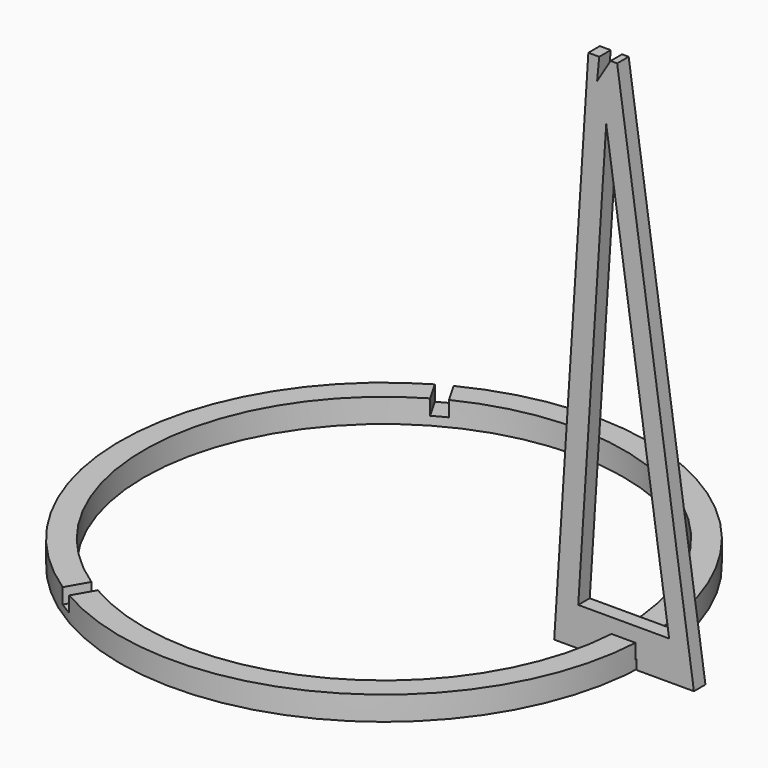
from build123d import *

# Parameters (mm, degrees)
F5_DEPTH = 3
F6_R     = 55
F6_R_2   = 50
F7_DEPTH = 5
F8_W     = 6.9784420547
F8_H     = 3.1
F9_DEPTH = 3.2


with BuildPart() as f5:
    # F4 (on Front) → F5 (new body)
    with BuildSketch(Plane.XZ):
        Polygon((47.2665503621, 110), (45, 110), (37.8812104464, 0), (49.8, 0), (49.8, 2), (55, 2), (55, 0), (67, 0), (51, 110), (49.6243909001, 110), (46.8244552612, 105.406075716), align=None)
        Polygon((61.8351592405, 8), (42.8892941961, 8), (48.7231474716, 98.1450809113), align=None, mode=Mode.SUBTRACT)
    extrude(amount=F5_DEPTH)


with BuildPart() as f7:
    # F6 (on Top) → F7 (new body)
    with BuildSketch(Plane.XY):
        Circle(F6_R)
        Circle(F6_R_2, mode=Mode.SUBTRACT)
    extrude(amount=F7_DEPTH)

    # F8 (on face) → F9 (cut)
    with BuildSketch(Plane.XY.offset(5)):
        with Locations((52.5480711023, -1.55)):
            Rectangle(F8_W, F8_H)
        Polygon((-28.0186460648, 48.5297185436), (-24.5294250375, 42.4862104453), (-21.8447462857, 44.0362104453), (-25.3339673131, 50.0797185436), align=None)
        Polygon((-28.0186460648, -48.5297185436), (-24.5294250375, -42.4862104453), (-27.2141037892, -40.9362104453), (-30.7033248166, -46.9797185436), align=None)
    extrude(amount=-F9_DEPTH, mode=Mode.SUBTRACT)


solid = Compound([f5.part, f7.part])
